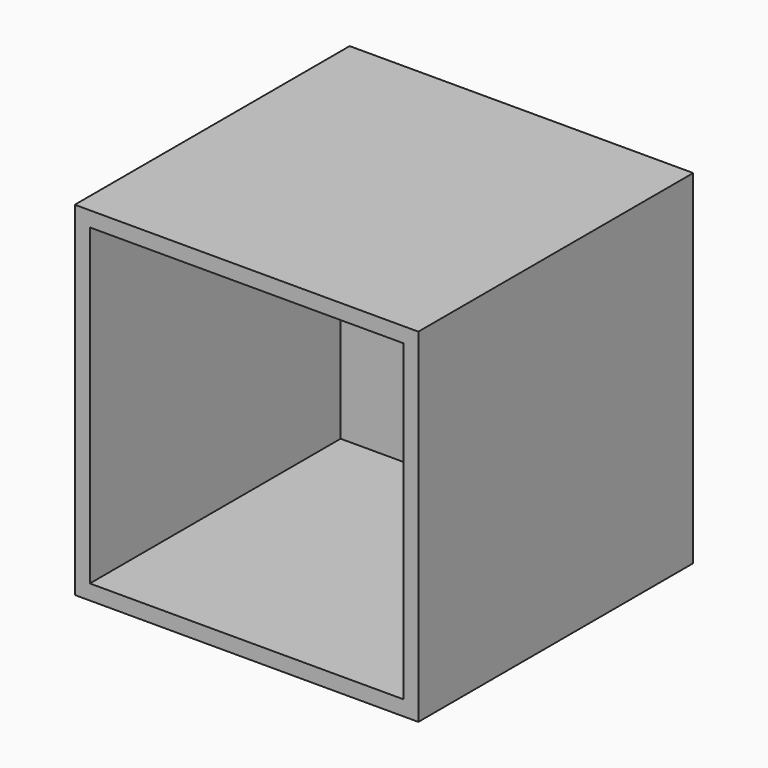
from build123d import *

# Parameters (mm, degrees)
F0_W         = 95
F0_H         = 95
F1_DEPTH     = 95
F2_W         = 86.6666666667
F2_H         = 86.6666666667
F3_DEPTH     = 86.6666666667
F4_TEXT_SIZE = 27.3501862668
F5_DEPTH     = 2.5


# Not quite as in the source:
# - Text() gives the source's letters only with a copy of the font that has no kerning and outlines rounded to 1/6400 em; it was checked with that copy


with BuildPart() as f1:
    # F0 (on Front) → F1 (new body)
    with BuildSketch(Plane.XZ):
        Rectangle(F0_W, F0_H)
    extrude(amount=F1_DEPTH)

    # F2 (on face) → F3 (cut)
    with BuildSketch(Plane.XZ.offset(95)):
        Rectangle(F2_W, F2_H)
    extrude(amount=-F3_DEPTH, mode=Mode.SUBTRACT)

    # F4 (on face) → F5 (join)
    with BuildSketch(Plane(origin=(-47.5, 0, 0), x_dir=(0, -1, 0), z_dir=(-1, 0, 0))):
        with Locations((17.3203833401, 19.2186273634)):
            Text('Ben', F4_TEXT_SIZE, font='Open Sans', text_align=(TextAlign.LEFT, TextAlign.BOTTOM))
    extrude(amount=F5_DEPTH)


solid = f1.part
